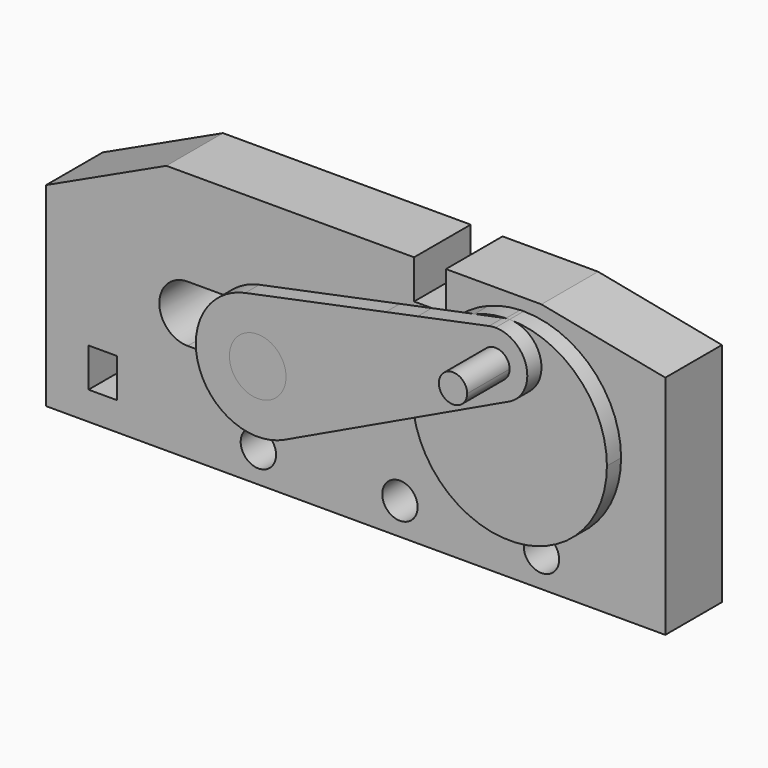
from build123d import *

# Parameters (mm, degrees)
F1_DEPTH       = 20
F2_W           = 8
F2_H           = 11
F2_R           = 5
F2_R_2         = 10
F3_DEPTH       = 20
F5_DEPTH       = 5
F5_DEPTH_BACK  = 25
F7_R           = 4.99999
F8_DEPTH       = 5
F9_DEPTH       = 25
F10_START      = 5
F10_DEPTH      = 5
F11_DEPTH      = 25
F11_DEPTH_BACK = 10
F12_DEPTH      = 25


# Not quite as in the source:
# - a fillet or chamfer is up to 0.001 mm smaller than in the source, because OpenCascade refuses the exact size


with BuildPart() as f1:
    # F0 (on Front) → F1 (new body)
    with BuildSketch(Plane.XZ):
        Polygon((0, 55), (0, 0), (175, 0), (175, 64), (140, 70.8544603773), (113, 70.8544603773), (113, 59.8544603773), (104, 59.8544603773), (104, 70.8544603773), (34, 70.8544603773), align=None)
    extrude(amount=F1_DEPTH)

    # F2 (on face) → F3 (cut, through all)
    with BuildSketch(Plane.XZ.offset(20)):
        with Locations((16, 13.5)):
            Rectangle(F2_W, F2_H)
        with Locations((60, 9)):
            Circle(F2_R)
        with BuildLine():
            Line((88, 44), (40, 44))
            ThreePointArc((40, 44), (32, 36), (40, 28))
            Line((40, 28), (88, 28))
            ThreePointArc((88, 28), (96, 36), (88, 44))
        make_face()
        with Locations((135, 40)):
            Circle(F2_R_2)
        with Locations((100, 9)):
            Circle(F2_R)
        with Locations((140, 9)):
            Circle(F2_R)
    extrude(amount=-F3_DEPTH, mode=Mode.SUBTRACT)


with BuildPart() as f5:
    # F4 (on face) → F5 (new body, two sides)
    with BuildSketch(Plane.XZ.offset(20)) as f5_sk:
        with BuildLine():
            ThreePointArc((148, 40), (146.0579755506, 46.8352890738), (140.8121266581, 51.6283783784))
            ThreePointArc((140.8121266581, 51.6283783784), (139.8774040705, 50.9362093146), (138.8612225529, 50.3703652975))
            Line((138.8612225529, 50.3703652975), (137.4433104674, 49.6969187869))
            ThreePointArc((137.4433104674, 49.6969187869), (142.8877469747, 46.1468241933), (145, 40))
            ThreePointArc((145, 40), (132.8316568043, 30.2379158073), (125.9403424429, 44.2335097671))
            Line((125.9403424429, 44.2335097671), (122.2377651401, 42.4749467432))
            ThreePointArc((122.2377651401, 42.4749467432), (133.7568292913, 27.0595778048), (148, 40))
        make_face()
        with BuildLine():
            ThreePointArc((138.8612225529, 50.3703652975), (139.8774040705, 50.9362093146), (140.8121266581, 51.6283783784))
            ThreePointArc((140.8121266581, 51.6283783784), (137.9858902425, 52.6524487535), (135, 53))
            Line((135, 53), (135, 50))
            ThreePointArc((135, 50), (136.2310183043, 49.9239404439), (137.4433104674, 49.6969187869))
            Line((137.4433104674, 49.6969187869), (138.8612225529, 50.3703652975))
        make_face()
        with BuildLine():
            Line((135, 50), (135, 53))
            ThreePointArc((135, 53), (126.7287941527, 50.0293147239), (122.2377651401, 42.4749467432))
            Line((122.2377651401, 42.4749467432), (125.9403424429, 44.2335097671))
            ThreePointArc((125.9403424429, 44.2335097671), (129.6304142465, 48.4360861088), (135, 50))
        make_face()
        with BuildLine():
            Line((135, 48.5364526865), (135, 50))
            ThreePointArc((135, 50), (129.6304142465, 48.4360861088), (125.9403424429, 44.2335097671))
            Line((125.9403424429, 44.2335097671), (135, 48.5364526865))
        make_face()
        with BuildLine():
            ThreePointArc((145, 40), (142.8877469747, 46.1468241933), (137.4433104674, 49.6969187869))
            Line((137.4433104674, 49.6969187869), (135, 48.5364526865))
            Line((135, 48.5364526865), (125.9403424429, 44.2335097671))
            ThreePointArc((125.9403424429, 44.2335097671), (132.8316568043, 30.2379158073), (145, 40))
        make_face()
        with BuildLine():
            Line((135, 48.5364526865), (137.4433104674, 49.6969187869))
            ThreePointArc((137.4433104674, 49.6969187869), (136.2310183043, 49.9239404439), (135, 50))
            Line((135, 50), (135, 48.5364526865))
        make_face()
    extrude(amount=F5_DEPTH)
    extrude(f5_sk.sketch, amount=-F5_DEPTH_BACK)

    # F6: cut F1
    add(f1.part, mode=Mode.SUBTRACT)

    # F7 (radius 5 in the source; OpenCascade refuses exactly that, so slightly less here)
    f7_edges = [f5.edges().sort_by_distance(p)[0] for p in [
        (135, 5, 27),
    ]]
    fillet(f7_edges, radius=F7_R)

    # F4 (on face) → F8 (join)
    with BuildSketch(Plane.XZ.offset(20)):
        with BuildLine():
            ThreePointArc((142.2400098005, 13.470162871), (156.8557803511, 23.3094378392), (162.5, 40))
            ThreePointArc((162.5, 40), (154.4454364826, 59.4454364826), (135, 67.5))
            ThreePointArc((135, 67.5), (143.4511713565, 61.5947863743), (140.8121266581, 51.6283783784))
            ThreePointArc((140.8121266581, 51.6283783784), (146.0579755506, 46.8352890738), (148, 40))
            ThreePointArc((148, 40), (133.7568292913, 27.0595778048), (122.2377651401, 42.4749467432))
            Line((122.2377651401, 42.4749467432), (107.8477760814, 35.6403284212))
            ThreePointArc((107.8477760814, 35.6403284212), (117.7276760177, 18.601008803), (136.4681544997, 12.5392184677))
            ThreePointArc((136.4681544997, 12.5392184677), (139.2038378059, 13.9362056036), (142.2400098005, 13.470162871))
        make_face()
        with BuildLine():
            ThreePointArc((140.8121266581, 51.6283783784), (143.4511713565, 61.5947863743), (135, 67.5))
            ThreePointArc((135, 67.5), (134.0885205875, 67.4537257765), (133.1864140644, 67.3153789513))
            Line((133.1864140644, 67.3153789513), (125.0755076463, 65.646723992))
            ThreePointArc((125.0755076463, 65.646723992), (111.1511705492, 53.6924553615), (107.8477760814, 35.6403284212))
            Line((107.8477760814, 35.6403284212), (122.2377651401, 42.4749467432))
            ThreePointArc((122.2377651401, 42.4749467432), (126.7287941527, 50.0293147239), (135, 53))
            ThreePointArc((135, 53), (137.9858902425, 52.6524487535), (140.8121266581, 51.6283783784))
        make_face()
        with BuildLine():
            ThreePointArc((139, 58.5), (137.8284271247, 55.6715728753), (135, 54.5))
            ThreePointArc((135, 54.5), (132.1715728753, 61.3284271247), (139, 58.5))
        make_face(mode=Mode.SUBTRACT)
        with BuildLine():
            Line((133.1864140644, 67.3153789513), (133.9944124644, 67.481608281))
            ThreePointArc((133.9944124644, 67.481608281), (129.458487419, 66.9358801288), (125.0755076463, 65.646723992))
            Line((125.0755076463, 65.646723992), (133.1864140644, 67.3153789513))
        make_face()
        with BuildLine():
            ThreePointArc((133.1864140644, 67.3153789513), (134.0885205875, 67.4537257765), (135, 67.5))
            ThreePointArc((135, 67.5), (134.4971221453, 67.4954016858), (133.9944124644, 67.481608281))
            Line((133.9944124644, 67.481608281), (133.1864140644, 67.3153789513))
        make_face()
        with BuildLine():
            ThreePointArc((136.4681544997, 12.5392184677), (139.3788920677, 12.8508691804), (142.2400098005, 13.470162871))
            ThreePointArc((142.2400098005, 13.470162871), (139.2038378059, 13.9362056036), (136.4681544997, 12.5392184677))
        make_face()
    extrude(amount=F8_DEPTH)


with BuildPart() as f9:
    # F4 (on face) → F9 (new body)
    with BuildSketch(Plane.XZ.offset(20)):
        with BuildLine():
            ThreePointArc((139, 58.5), (132.1715728753, 61.3284271247), (135, 54.5))
            ThreePointArc((135, 54.5), (137.8284271247, 55.6715728753), (139, 58.5))
        make_face()
    extrude(amount=F9_DEPTH)


with BuildPart() as f10:
    # F4 (on face) → F10 (new body)
    with BuildSketch(Plane.XZ.offset(20).offset(F10_START)):
        with BuildLine():
            ThreePointArc((140.8121266581, 51.6283783784), (143.4511713565, 61.5947863743), (135, 67.5))
            ThreePointArc((135, 67.5), (134.0885205875, 67.4537257765), (133.1864140644, 67.3153789513))
            Line((133.1864140644, 67.3153789513), (125.0755076463, 65.646723992))
            ThreePointArc((125.0755076463, 65.646723992), (111.1511705492, 53.6924553615), (107.8477760814, 35.6403284212))
            Line((107.8477760814, 35.6403284212), (122.2377651401, 42.4749467432))
            ThreePointArc((122.2377651401, 42.4749467432), (126.7287941527, 50.0293147239), (135, 53))
            ThreePointArc((135, 53), (137.9858902425, 52.6524487535), (140.8121266581, 51.6283783784))
        make_face()
        with BuildLine():
            ThreePointArc((139, 58.5), (137.8284271247, 55.6715728753), (135, 54.5))
            ThreePointArc((135, 54.5), (132.1715728753, 61.3284271247), (139, 58.5))
        make_face(mode=Mode.SUBTRACT)
        with BuildLine():
            ThreePointArc((138.8612225529, 50.3703652975), (139.8774040705, 50.9362093146), (140.8121266581, 51.6283783784))
            ThreePointArc((140.8121266581, 51.6283783784), (137.9858902425, 52.6524487535), (135, 53))
            Line((135, 53), (135, 50))
            ThreePointArc((135, 50), (136.2310183043, 49.9239404439), (137.4433104674, 49.6969187869))
            Line((137.4433104674, 49.6969187869), (138.8612225529, 50.3703652975))
        make_face()
        with BuildLine():
            ThreePointArc((107.8477760814, 35.6403284212), (111.1511705492, 53.6924553615), (125.0755076463, 65.646723992))
            Line((125.0755076463, 65.646723992), (113, 63.1624325107))
            Line((113, 63.1624325107), (113, 59.8544603773))
            Line((113, 59.8544603773), (104, 59.8544603773))
            Line((104, 59.8544603773), (104, 61.3108645282))
            Line((104, 61.3108645282), (64.2884421212, 53.1410146274))
            ThreePointArc((64.2884421212, 53.1410146274), (57.231655846, 49.9372094187), (52.2504768019, 44))
            Line((52.2504768019, 44), (58.5414022207, 44))
            Line((58.5414022207, 44), (67.8148592182, 44))
            Line((67.8148592182, 44), (76.3124004006, 44))
            Line((76.3124004006, 44), (88, 44))
            ThreePointArc((88, 44), (96, 36), (88, 28))
            Line((88, 28), (76.3124004006, 28))
            Line((76.3124004006, 28), (67.8148592182, 28))
            Line((67.8148592182, 28), (58.5414022207, 28))
            Line((58.5414022207, 28), (52.2504768019, 28))
            ThreePointArc((52.2504768019, 28), (62.2053726379, 19.4234002188), (75.32279196, 20.1923769673))
            Line((75.32279196, 20.1923769673), (107.8477760814, 35.6403284212))
        make_face()
        with BuildLine():
            Line((135, 50), (135, 53))
            ThreePointArc((135, 53), (126.7287941527, 50.0293147239), (122.2377651401, 42.4749467432))
            Line((122.2377651401, 42.4749467432), (125.9403424429, 44.2335097671))
            ThreePointArc((125.9403424429, 44.2335097671), (129.6304142465, 48.4360861088), (135, 50))
        make_face()
        Polygon((113, 59.8544603773), (113, 63.1624325107), (104, 61.3108645282), (104, 59.8544603773), align=None)
        with BuildLine():
            Line((135, 48.5364526865), (137.4433104674, 49.6969187869))
            ThreePointArc((137.4433104674, 49.6969187869), (136.2310183043, 49.9239404439), (135, 50))
            Line((135, 50), (135, 48.5364526865))
        make_face()
        with BuildLine():
            Line((135, 48.5364526865), (135, 50))
            ThreePointArc((135, 50), (129.6304142465, 48.4360861088), (125.9403424429, 44.2335097671))
            Line((125.9403424429, 44.2335097671), (135, 48.5364526865))
        make_face()
        with BuildLine():
            ThreePointArc((52.2504768019, 44), (50.3148592182, 36), (52.2504768019, 28))
            Line((52.2504768019, 28), (58.5414022207, 28))
            Line((58.5414022207, 28), (58.5414022207, 44))
            Line((58.5414022207, 44), (52.2504768019, 44))
        make_face()
        with BuildLine():
            Line((58.5414022207, 44), (58.5414022207, 28))
            Line((58.5414022207, 28), (67.8148592182, 28))
            ThreePointArc((67.8148592182, 28), (59.8148592182, 36), (67.8148592182, 44))
            Line((67.8148592182, 44), (58.5414022207, 44))
        make_face()
        with BuildLine():
            ThreePointArc((75.8148592182, 36), (73.4717134677, 30.3431457505), (67.8148592182, 28))
            Line((67.8148592182, 28), (76.3124004006, 28))
            Line((76.3124004006, 28), (76.3124004006, 44))
            Line((76.3124004006, 44), (67.8148592182, 44))
            ThreePointArc((67.8148592182, 44), (73.4717134677, 41.6568542495), (75.8148592182, 36))
        make_face()
        with BuildLine():
            Line((76.3124004006, 44), (76.3124004006, 28))
            Line((76.3124004006, 28), (88, 28))
            ThreePointArc((88, 28), (96, 36), (88, 44))
            Line((88, 44), (76.3124004006, 44))
        make_face()
    extrude(amount=F10_DEPTH)


with BuildPart() as f11:
    # F4 (on face) → F11 (new body, two sides)
    with BuildSketch(Plane.XZ.offset(20)) as f11_sk:
        with BuildLine():
            ThreePointArc((67.8148592182, 44), (59.8148592182, 36), (67.8148592182, 28))
            ThreePointArc((67.8148592182, 28), (73.4717134677, 30.3431457505), (75.8148592182, 36))
            ThreePointArc((75.8148592182, 36), (73.4717134677, 41.6568542495), (67.8148592182, 44))
        make_face()
    extrude(amount=-F11_DEPTH)
    extrude(f11_sk.sketch, amount=F11_DEPTH_BACK)

    # F4 (on face) → F12 (join)
    with BuildSketch(Plane.XZ.offset(20)):
        with BuildLine():
            Line((58.5414022207, 44), (58.5414022207, 28))
            Line((58.5414022207, 28), (67.8148592182, 28))
            ThreePointArc((67.8148592182, 28), (59.8148592182, 36), (67.8148592182, 44))
            Line((67.8148592182, 44), (58.5414022207, 44))
        make_face()
        with BuildLine():
            ThreePointArc((75.8148592182, 36), (73.4717134677, 30.3431457505), (67.8148592182, 28))
            Line((67.8148592182, 28), (76.3124004006, 28))
            Line((76.3124004006, 28), (76.3124004006, 44))
            Line((76.3124004006, 44), (67.8148592182, 44))
            ThreePointArc((67.8148592182, 44), (73.4717134677, 41.6568542495), (75.8148592182, 36))
        make_face()
    extrude(amount=-F12_DEPTH)


solid = Compound([f1.part, f5.part, f9.part, f10.part, f11.part])
